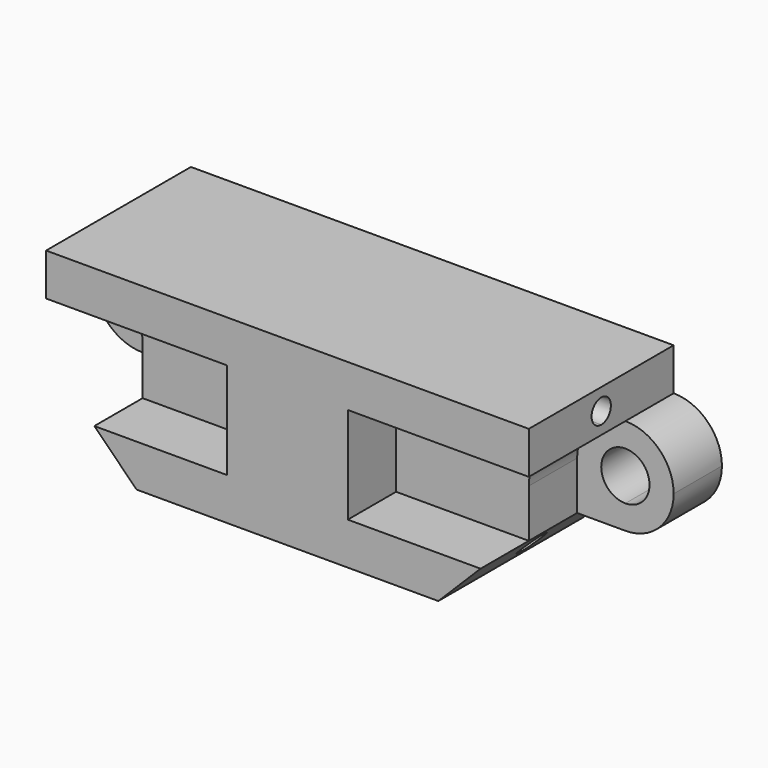
from build123d import *

# Parameters (mm, degrees)
F0_W        = 11
F0_H        = 4
F0_W_2      = 10
F1_DEPTH    = 10
F2_DEPTH    = 5
F3_DEPTH    = 15
F5_DEPTH    = 40
F6_T1_DEPTH = 33.0017809158


# Not quite as in the source:
# - a fillet or chamfer that OpenCascade refuses, or shapes differently, is made with other operations: its cross-section is extruded or revolved along the edge and cut away or added


with BuildPart() as f1:
    # F0 (on Front) → F1 (new body)
    with BuildSketch(Plane.XZ):
        Polygon((-5, 4), (5, 4), (20, 4), (20, 7.5), (-20, 7.5), (-20, 4), align=None)
        with BuildLine():
            Line((-5, 0), (-5, 4))
            Line((-5, 4), (-20, 4))
            ThreePointArc((-20, 4), (-17.1715728753, 2.8284271247), (-16, 0))
            Line((-16, 0), (-5, 0))
        make_face()
        with Locations((-10.5, -2)):
            Rectangle(F0_W, F0_H)
        Polygon((16, -4), (5, -4), (-5, -4), (-16, -4), (-16, -7.5), (16, -7.5), align=None)
        with Locations((0, -2)):
            Rectangle(F0_W_2, F0_H)
        with Locations((0, 2)):
            Rectangle(F0_W_2, F0_H)
        with BuildLine():
            Line((20, 4), (5, 4))
            Line((5, 4), (5, 0))
            Line((5, 0), (16, 0))
            ThreePointArc((16, 0), (17.1715728753, 2.8284271247), (20, 4))
        make_face()
        with Locations((10.5, -2)):
            Rectangle(F0_W, F0_H)
    extrude(amount=F1_DEPTH)

    # F0 (on Front) → F2 (join)
    with BuildSketch(Plane.XZ):
        with BuildLine():
            Line((-20, 2), (-20, 4))
            ThreePointArc((-20, 4), (-24, 0), (-20, -4))
            Line((-20, -4), (-20, -2))
            ThreePointArc((-20, -2), (-22, 0), (-20, 2))
        make_face()
        with BuildLine():
            ThreePointArc((-16, 0), (-17.1715728753, 2.8284271247), (-20, 4))
            Line((-20, 4), (-20, 2))
            ThreePointArc((-20, 2), (-18.5857864376, 1.4142135624), (-18, 0))
            ThreePointArc((-18, 0), (-18.5857864376, -1.4142135624), (-20, -2))
            Line((-20, -2), (-20, -4))
            ThreePointArc((-20, -4), (-17.1715728753, -2.8284271247), (-16, 0))
        make_face()
        with BuildLine():
            Line((-16, -4), (-16, 0))
            ThreePointArc((-16, 0), (-17.1715728753, -2.8284271247), (-20, -4))
            Line((-20, -4), (-16, -4))
        make_face()
        with BuildLine():
            ThreePointArc((20, -4), (17.1715728753, -2.8284271247), (16, 0))
            Line((16, 0), (16, -4))
            Line((16, -4), (20, -4))
        make_face()
        with BuildLine():
            Line((20, 2), (20, 4))
            ThreePointArc((20, 4), (17.1715728753, 2.8284271247), (16, 0))
            ThreePointArc((16, 0), (17.1715728753, -2.8284271247), (20, -4))
            Line((20, -4), (20, -2))
            ThreePointArc((20, -2), (18, 0), (20, 2))
        make_face()
        with BuildLine():
            ThreePointArc((24, 0), (22.8284271247, 2.8284271247), (20, 4))
            Line((20, 4), (20, 2))
            ThreePointArc((20, 2), (21.4142135624, 1.4142135624), (22, 0))
            ThreePointArc((22, 0), (21.4142135624, -1.4142135624), (20, -2))
            Line((20, -2), (20, -4))
            ThreePointArc((20, -4), (22.8284271247, -2.8284271247), (24, 0))
        make_face()
    extrude(amount=F2_DEPTH)

    # F0 (on Front) → F3 (join)
    with BuildSketch(Plane.XZ):
        Polygon((16, -4), (5, -4), (-5, -4), (-16, -4), (-16, -7.5), (16, -7.5), align=None)
        with Locations((0, -2)):
            Rectangle(F0_W_2, F0_H)
        with Locations((0, 2)):
            Rectangle(F0_W_2, F0_H)
        Polygon((-5, 4), (5, 4), (20, 4), (20, 7.5), (-20, 7.5), (-20, 4), align=None)
    extrude(amount=F3_DEPTH)

    # F4 (on face) → F5 (cut)
    with BuildSketch(Plane(origin=(-20, 0, 0), x_dir=(0, -1, 0), z_dir=(-1, 0, 0))):
        with BuildLine():
            ThreePointArc((8.5, -5.75), (8.2071067812, -5.0428932188), (7.5, -4.75))
            Line((7.5, -4.75), (7.5, -6.75))
            ThreePointArc((7.5, -6.75), (8.2071067812, -6.4571067812), (8.5, -5.75))
        make_face()
        with BuildLine():
            Line((7.5, -6.75), (7.5, -4.75))
            ThreePointArc((7.5, -4.75), (6.5, -5.75), (7.5, -6.75))
        make_face()
        with BuildLine():
            ThreePointArc((7.5, 6.75), (6.5, 5.75), (7.5, 4.75))
            Line((7.5, 4.75), (7.5, 6.75))
        make_face()
        with BuildLine():
            Line((7.5, 6.75), (7.5, 4.75))
            ThreePointArc((7.5, 4.75), (8.2071067812, 5.0428932188), (8.5, 5.75))
            ThreePointArc((8.5, 5.75), (8.2071067812, 6.4571067812), (7.5, 6.75))
        make_face()
    extrude(amount=-F5_DEPTH, mode=Mode.SUBTRACT)

    # F6: chamfer of 3.5 on 2 edges, made by hand

    # F6_s2 → F6_t1 (cut)
    with BuildSketch(Plane.XZ.offset(-9.0008904579)):
        Polygon((-16, -4), (-12.5, -7.5), (-16, -7.5), align=None)
        Polygon((16, -4), (12.5, -7.5), (16, -7.5), align=None)
    extrude(amount=F6_T1_DEPTH, mode=Mode.SUBTRACT)


solid = f1.part
